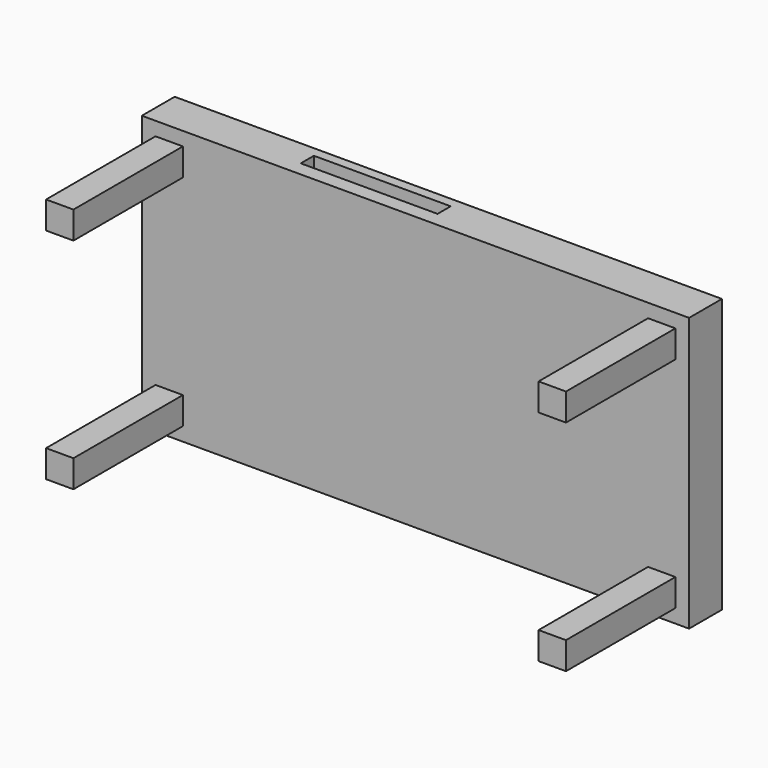
from build123d import *

# Parameters (mm, degrees)
F0_W     = 200
F0_H     = 100
F1_DEPTH = 15
F2_W     = 10
F2_H     = 10
F3_DEPTH = 50
F4_W     = 50
F4_H     = 6
F5_DEPTH = 10


# Not quite as in the source:
# - a feature names something its author has since deleted; it is built from what else it names


with BuildPart() as f1:
    # F0 (on Front) → F1 (new body)
    with BuildSketch(Plane.XZ):
        with Locations((46.1999992281, 49.9613083565)):
            Rectangle(F0_W, F0_H)
    extrude(amount=F1_DEPTH)

    # F2 (on face) → F3 (join)
    with BuildSketch(Plane.XZ.offset(15)):
        with Locations((-43.8000007719, 89.9613083565)):
            Rectangle(F2_W, F2_H)
        with Locations((-43.8000007719, 9.9613083565)):
            Rectangle(F2_W, F2_H)
        with Locations((136.1999992281, 89.9613083565)):
            Rectangle(F2_W, F2_H)
        with Locations((136.1999992281, 9.9613083565)):
            Rectangle(F2_W, F2_H)
    extrude(amount=F3_DEPTH)

    # F4 (on face) → F5 (cut, symmetric)
    with BuildSketch(Plane.XY.offset(94.9613083565)):
        with Locations((25, -6.6546534393)):
            Rectangle(F4_W, F4_H)
    extrude(amount=F5_DEPTH, both=True, mode=Mode.SUBTRACT)


solid = f1.part
